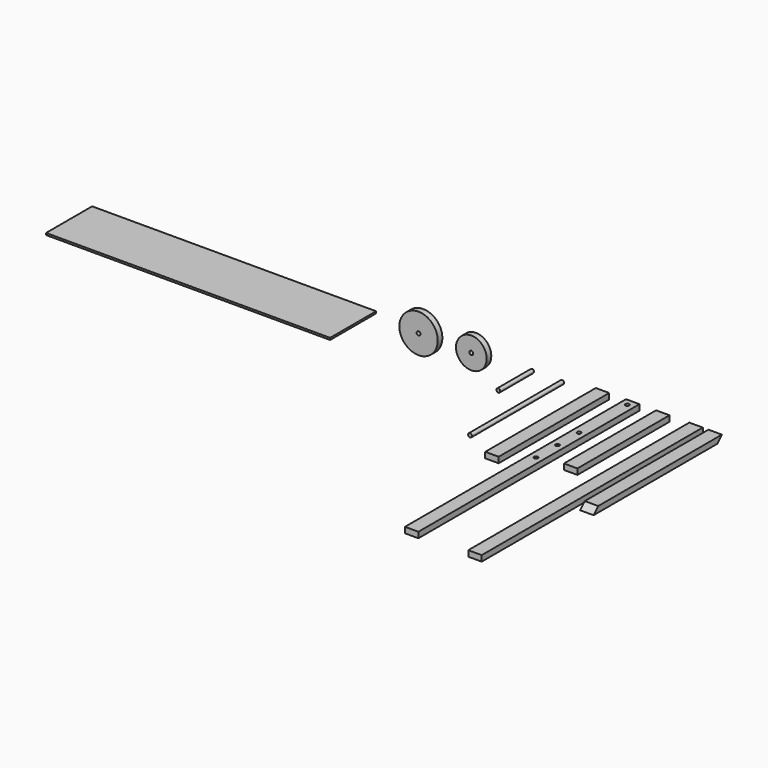
from build123d import *

# Parameters (mm, degrees)
F0_W      = 88.9
F0_H      = 38.1
F1_DEPTH  = 914.4
F2_DEPTH  = 1828.8
F3_DEPTH  = 762
F5_D      = 25.4
F6_W      = 1879.6
F6_H      = 381
F7_DEPTH  = 12.7
F8_R      = 12.7
F9_DEPTH  = 762
F10_DEPTH = 279.4
F11_R     = 101.6
F12_DEPTH = 38.1
F11_R_2   = 127
F13_DEPTH = 38.1
F14_D     = 25.4
F15_D     = 25.4
F16_W     = 88.9
F16_H     = 38.1
F17_DEPTH = 1061.72
F18_SIZE  = 38.09999


# Not quite as in the source:
# - a fillet or chamfer is up to 0.001 mm smaller than in the source, because OpenCascade refuses the exact size


with BuildPart() as f1:
    # F0 (on Front) → F1 (new body)
    with BuildSketch(Plane.XZ):
        with Locations((44.45, 19.05)):
            Rectangle(F0_W, F0_H)
    extrude(amount=F1_DEPTH)


with BuildPart() as f2:
    # F0 (on Front) → F2 (new body)
    with BuildSketch(Plane.XZ):
        with Locations((244.851688537, 19.05)):
            Rectangle(F0_W, F0_H)
    extrude(amount=F2_DEPTH)

    # F5 (through all)
    with Locations(Plane.XY.offset(38.1)):
        with Locations((244.851688537, -44.45), (244.851688537, -444.5), (244.851688537, -622.3), (244.851688537, -800.1)):
            Hole(F5_D / 2)


with BuildPart() as f2b:
    # F0 (on Front) → F2, piece 2 (new body)
    with BuildSketch(Plane.XZ):
        with Locations((663.7364707975, 19.05)):
            Rectangle(F0_W, F0_H)
    extrude(amount=F2_DEPTH)


with BuildPart() as f3:
    # F0 (on Front) → F3 (new body)
    with BuildSketch(Plane.XZ):
        with Locations((443.7466020195, 19.05)):
            Rectangle(F0_W, F0_H)
    extrude(amount=F3_DEPTH)


with BuildPart() as f7:
    # F6 (on Top) → F7 (new body)
    with BuildSketch(Plane.XY):
        with Locations((-2393.1029083252, -190.5)):
            Rectangle(F6_W, F6_H)
    extrude(amount=F7_DEPTH)


with BuildPart() as f9:
    # F8 (on Front) → F9 (new body)
    with BuildSketch(Plane.XZ):
        with Locations((-222.2214488977, 0)):
            Circle(F8_R)
    extrude(amount=F9_DEPTH)


with BuildPart() as f10:
    # F8 (on Front) → F10 (new body)
    with BuildSketch(Plane.XZ):
        with Locations((-421.2695658207, 0)):
            Circle(F8_R)
    extrude(amount=F10_DEPTH)


with BuildPart() as f12:
    # F11 (on Front) → F12 (new body)
    with BuildSketch(Plane.XZ):
        with Locations((-792.9399567111, 0)):
            Circle(F11_R)
    extrude(amount=F12_DEPTH)

    # F14 (through all)
    with Locations(Plane(origin=(0, 0, 0), x_dir=(1, 0, 0), z_dir=(0, 1, 0))):
        with Locations((-792.9399567111, 0), (-1142.1980857849, 0)):
            Hole(F14_D / 2)


with BuildPart() as f13:
    # F11 (on Front) → F13 (new body)
    with BuildSketch(Plane.XZ):
        with Locations((-1142.1980857849, 0)):
            Circle(F11_R_2)
    extrude(amount=F13_DEPTH)

    # F15 (through all)
    with Locations(Plane(origin=(0, 0, 0), x_dir=(1, 0, 0), z_dir=(0, 1, 0))):
        with Locations((-1142.1980857849, 0)):
            Hole(F15_D / 2)


with BuildPart() as f17:
    # F16 (on Front) → F17 (new body)
    with BuildSketch(Plane.XZ):
        with Locations((790.4931433541, 19.05)):
            Rectangle(F16_W, F16_H)
    extrude(amount=F17_DEPTH)

    # F18 (size 38.1 in the source; OpenCascade refuses exactly that, so slightly less here)
    f18_edges = [f17.edges().sort_by_distance(p)[0] for p in [
        (790.493143, -1061.72, 38.1),
        (790.493143, 0, 0),
    ]]
    chamfer(f18_edges, length=F18_SIZE)


solid = Compound([f1.part, f2.part, f2b.part, f3.part, f7.part, f9.part, f10.part, f12.part, f13.part, f17.part])
